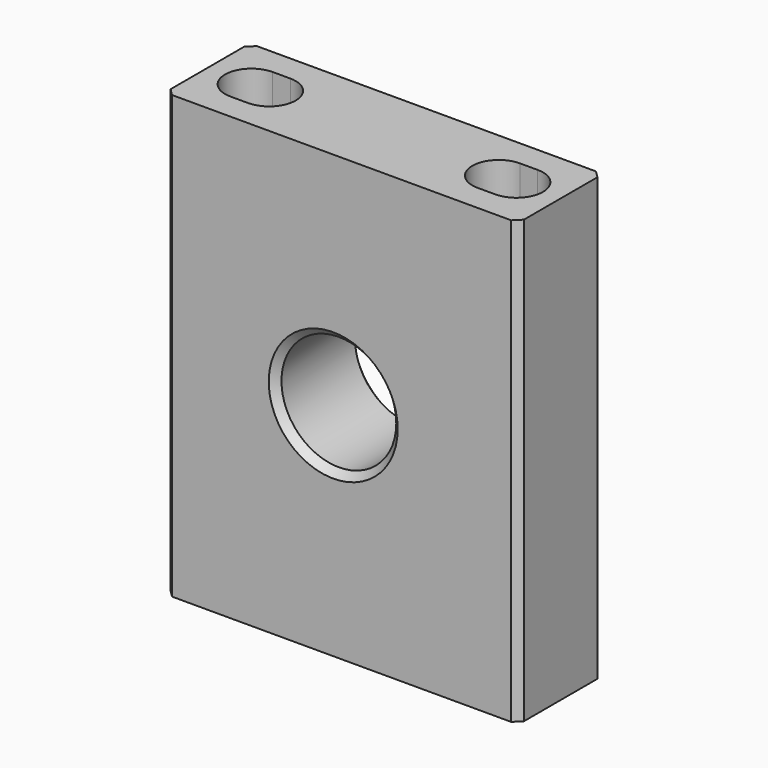
from build123d import *

# Parameters (mm, degrees)
F0_W     = 40
F0_H     = 12
F1_DEPTH = 50
F3_DEPTH = 55
F4_R     = 6.5
F5_DEPTH = 13
F6_SIZE  = 0.8


# Not quite as in the source:
# - a feature names something its author has since deleted; it is built from what else it names


with BuildPart() as f1:
    # F0 (on Top) → F1 (new body)
    with BuildSketch(Plane.XY):
        with Locations((-12.258, 6)):
            Rectangle(F0_W, F0_H)
    extrude(amount=F1_DEPTH)

    # F2 (on face) → F3 (cut)
    with BuildSketch(Plane.XY.offset(50)):
        with BuildLine():
            Line((-25.258, 9), (-27.258, 9))
            ThreePointArc((-27.258, 9), (-30.258, 6), (-27.258, 3))
            Line((-27.258, 3), (-25.258, 3))
            ThreePointArc((-25.258, 3), (-22.258, 6), (-25.258, 9))
        make_face()
        with BuildLine():
            Line((0.742, 3), (2.742, 3))
            ThreePointArc((2.742, 3), (5.742, 6), (2.742, 9))
            Line((2.742, 9), (0.742, 9))
            ThreePointArc((0.742, 9), (-2.258, 6), (0.742, 3))
        make_face()
    extrude(amount=-F3_DEPTH, mode=Mode.SUBTRACT)

    # F4 (on face) → F5 (cut)
    with BuildSketch(Plane.XZ):
        with Locations((-13.208, 25)):
            Circle(F4_R)
    extrude(amount=-F5_DEPTH, mode=Mode.SUBTRACT)

    # F6
    f6_edges = [f1.edges().sort_by_distance(p)[0] for p in [
        (7.742, 0, 25),
        (-32.258, 12, 25),
        (-32.258, 0, 25),
        (-19.708, 12, 25),
        (-19.708, 0, 25),
        (7.742, 12, 25),
    ]]
    chamfer(f6_edges, length=F6_SIZE)


solid = f1.part
